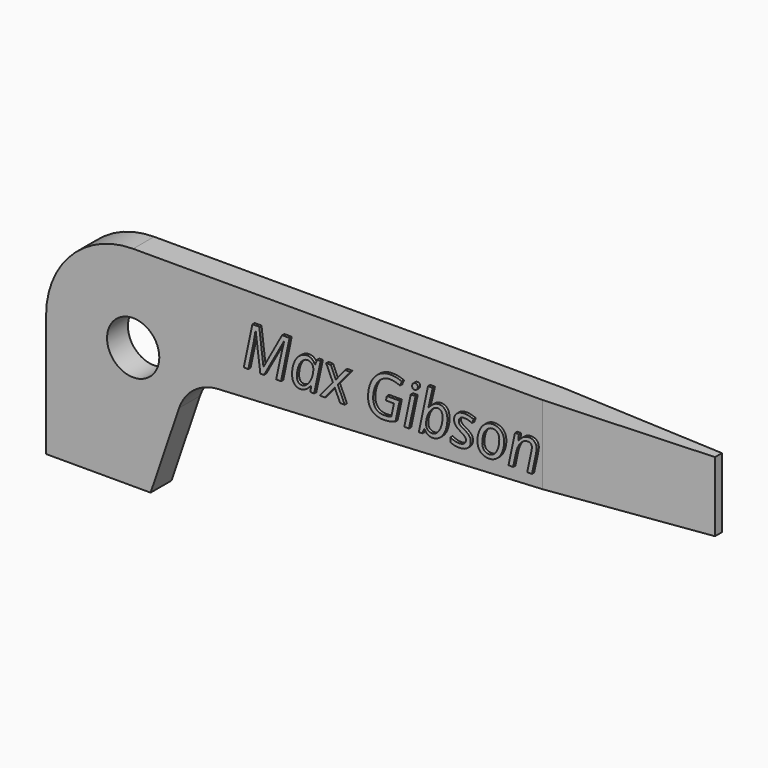
from build123d import *

# Parameters (mm, degrees)
F1_DEPTH     = 2.38125
F2_R         = 2.38125
F3_DEPTH     = 25.4
F5_DEPTH     = 25.4
F6_TEXT_SIZE = 5.2159044167
F7_DEPTH     = 0.254


# Not quite as in the source:
# - Text() gives the source's letters only with a copy of the font that has no kerning and outlines rounded to 1/6400 em; it was checked with that copy


with BuildPart() as f1:
    # F0 (on Front) → F1 (new body)
    with BuildSketch(Plane.XZ):
        with BuildLine():
            Line((60.325, 19.05), (7.9375, 19.05))
            ThreePointArc((7.9375, 19.05), (2.3248399243, 16.7251600757), (0, 11.1125))
            Line((0, 11.1125), (0, 0))
            Line((0, 0), (9.525, 0))
            Line((9.525, 0), (12.1173647876, 7.6271664624))
            ThreePointArc((12.1173647876, 7.6271664624), (13.4786145605, 9.5135918491), (15.6631963617, 10.3130942181))
            Line((15.6631963617, 10.3130942181), (60.325, 12.7))
            Line((60.325, 12.7), (60.325, 19.05))
        make_face()
    extrude(amount=F1_DEPTH)

    # F2 (on face) → F3 (cut)
    with BuildSketch(Plane.XZ.offset(2.38125)):
        with Locations((7.9375, 11.1125)):
            Circle(F2_R)
    extrude(amount=-F3_DEPTH, mode=Mode.SUBTRACT)

    # F4 (on face) → F5 (cut)
    with BuildSketch(Plane.XY.offset(19.05)):
        Polygon((60.325, -2.38125), (60.325, -1.5875), (45.24375, -2.38125), align=None)
        Polygon((60.325, 0), (45.24375, 0), (60.325, -0.79375), align=None)
    extrude(amount=-F5_DEPTH, mode=Mode.SUBTRACT)

    # F6 (on face) → F7 (join)
    with BuildSketch(Plane.XZ.offset(2.38125)):
        with Locations((18.007764109, 12.9735087976)):
            Text('Max Gibson', F6_TEXT_SIZE, font='Open Sans', font_style=FontStyle.ITALIC, text_align=(TextAlign.LEFT, TextAlign.BOTTOM))
    extrude(amount=F7_DEPTH)


solid = f1.part
